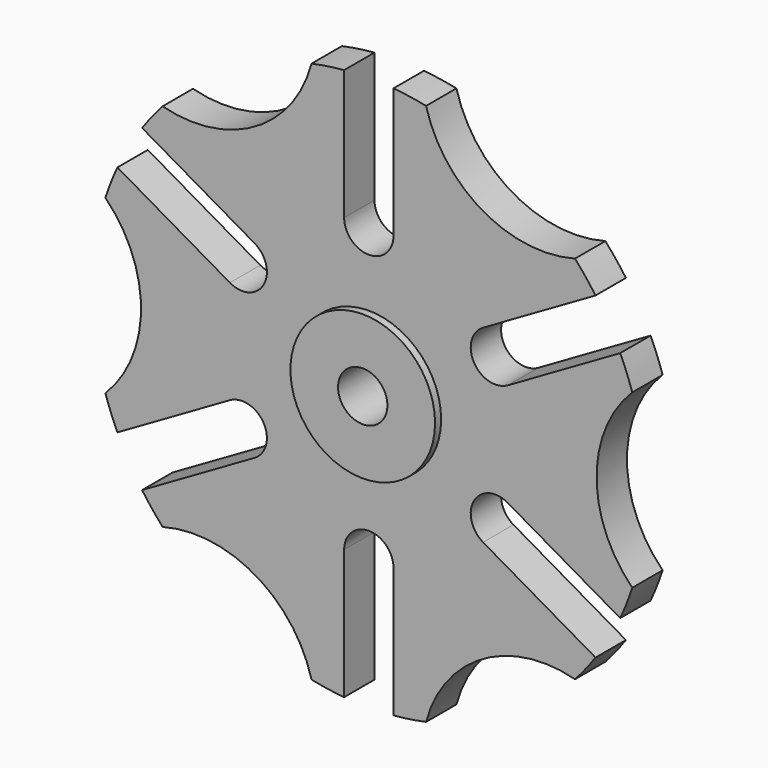
from build123d import *

# Parameters (mm, degrees)
F1_R            = 73
F2_DEPTH        = 5
F4_DEPTH        = 5.001
F4_DEPTH_BACK   = 5.001
F4_COPIES_COUNT = 6
F6_R            = 32
F7_DEPTH        = 5.001
F7_DEPTH_BACK   = 5.001
F7_COPIES_COUNT = 6
F8_R            = 19.05
F9_DEPTH        = 7
F10_R           = 6.5
F11_DEPTH       = 14.001


# Not quite as in the source:
# - a pattern or mirror of a feature is missing from the dataset's text; its kind, count and spacing are read off the source's solid


with BuildPart() as f2:
    # F1 (on Front) → F2 (new body, symmetric)
    with BuildSketch(Plane.XZ):
        Circle(F1_R)
    extrude(amount=F2_DEPTH, both=True)

    # F3 (on Front) → F4 (cut, two sides)
    with BuildSketch(Plane.XZ) as f4_sk:
        with BuildLine():
            Line((-6.5, 95.5425653795), (-6.5, 38.5))
            ThreePointArc((-6.5, 38.5), (0, 32), (6.5, 38.5))
            Line((6.5, 38.5), (6.5, 95.5425653795))
            Line((6.5, 95.5425653795), (-6.5, 95.5425653795))
        make_face()
    f4 = extrude(amount=-F4_DEPTH, mode=Mode.SUBTRACT) + extrude(f4_sk.sketch, amount=F4_DEPTH_BACK, mode=Mode.SUBTRACT)

    # F4_copies: F4 ×6 about axis
    f4_copies_axis = Axis((0, 0, 0), (0, 1, 0))
    for i in range(1, F4_COPIES_COUNT):
        add(f4.rotate(f4_copies_axis, i * 360 / F4_COPIES_COUNT), mode=Mode.SUBTRACT)

    # F6 (on Front) → F7 (cut, two sides)
    with BuildSketch(Plane.XZ) as f7_sk:
        with Locations((46, 79.6743371482)):
            Circle(F6_R)
    f7 = extrude(amount=-F7_DEPTH, mode=Mode.SUBTRACT) + extrude(f7_sk.sketch, amount=F7_DEPTH_BACK, mode=Mode.SUBTRACT)

    # F7_copies: F7 ×6 about axis
    f7_copies_axis = Axis((0, 0, 0), (0, 1, 0))
    for i in range(1, F7_COPIES_COUNT):
        add(f7.rotate(f7_copies_axis, i * 360 / F7_COPIES_COUNT), mode=Mode.SUBTRACT)

    # F8 (on Front) → F9 (join, symmetric)
    with BuildSketch(Plane.XZ):
        Circle(F8_R)
    extrude(amount=F9_DEPTH, both=True)

    # F10 (on face) → F11 (cut, through all)
    with BuildSketch(Plane(origin=(0, 7, 0), x_dir=(-1, 0, 0), z_dir=(0, 1, 0))):
        Circle(F10_R)
    extrude(amount=-F11_DEPTH, mode=Mode.SUBTRACT)


solid = f2.part
